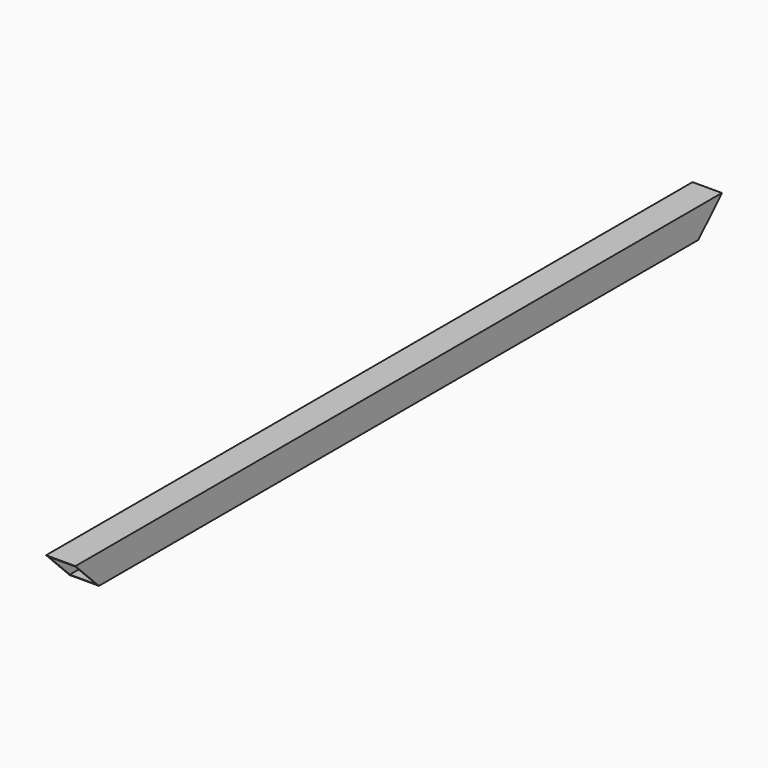
from build123d import *

# Parameters (mm, degrees)
F0_W        = 40
F0_H        = 40
F1_DEPTH    = 1100
F2_W        = 36
F2_H        = 36
F3_DEPTH    = 1100.001
F4_T1_DEPTH = 245.7346390373


# Not quite as in the source:
# - a fillet or chamfer that OpenCascade refuses, or shapes differently, is made with other operations: its cross-section is extruded or revolved along the edge and cut away or added


with BuildPart() as f1:
    # F0 (on Front) → F1 (new body)
    with BuildSketch(Plane.XZ):
        with Locations((20, 20)):
            Rectangle(F0_W, F0_H)
    extrude(amount=F1_DEPTH)

    # F2 (on face) → F3 (cut, through all)
    with BuildSketch(Plane.XZ.offset(1100)):
        with Locations((20, 20)):
            Rectangle(F2_W, F2_H)
    extrude(amount=-F3_DEPTH, mode=Mode.SUBTRACT)

    # F4: chamfer of 40 on 2 edges, made by hand

    # F4_s2 → F4_t1 (cut)
    with BuildSketch(Plane.YZ.offset(-102.8673195186)):
        Polygon((-1060, 0), (-1100, 40), (-1100, 0), align=None)
        Polygon((-40, 0), (0, 40), (0, 0), align=None)
    extrude(amount=F4_T1_DEPTH, mode=Mode.SUBTRACT)


solid = f1.part
